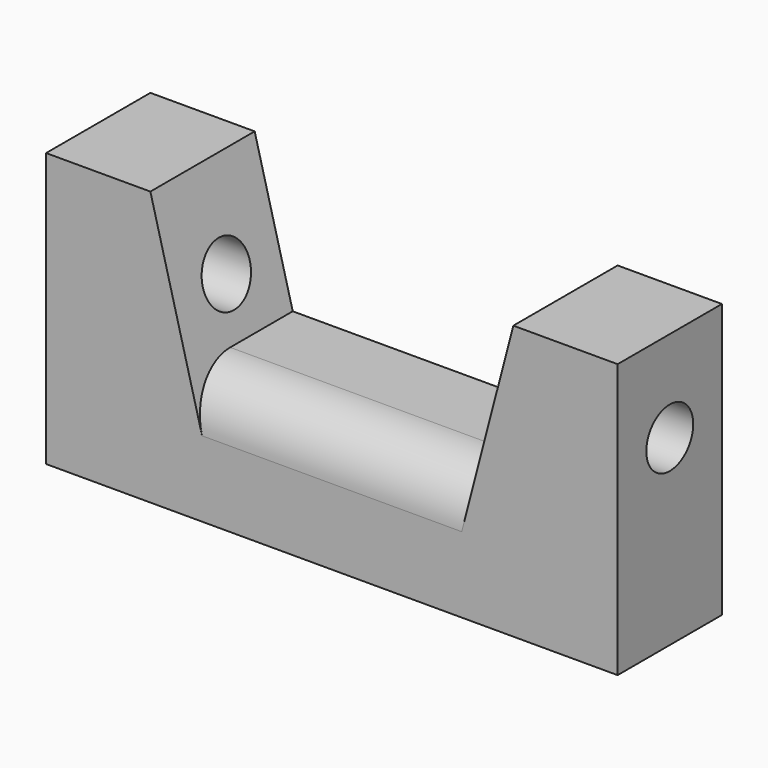
from build123d import *

# Parameters (mm, degrees)
F1_DEPTH = 31.75
F3_D     = 14.2875
F4_R     = 12.7


# Not quite as in the source:
# - a length typed as a fraction of an inch, garbled in the dataset ("3 / 203.2 mm" for 3/8 in), is restored


with BuildPart() as f1:
    # F0 (on Front) → F1 (new body)
    with BuildSketch(Plane.XZ):
        Polygon((0, 66.675), (0, 0), (139.192, 0), (139.192, 66.675), (113.792, 66.675), (104.521, 31.115), (34.671, 31.115), (25.4, 66.675), align=None)
    extrude(amount=F1_DEPTH)

    # F3 (through all)
    with Locations(Plane.YZ.offset(139.192)):
        with Locations((-15.875, 44.45)):
            Hole(F3_D / 2)

    # F4
    f4_edges = [f1.edges().sort_by_distance(p)[0] for p in [
        (69.596, -31.75, 31.115),
    ]]
    fillet(f4_edges, radius=F4_R)


solid = f1.part
